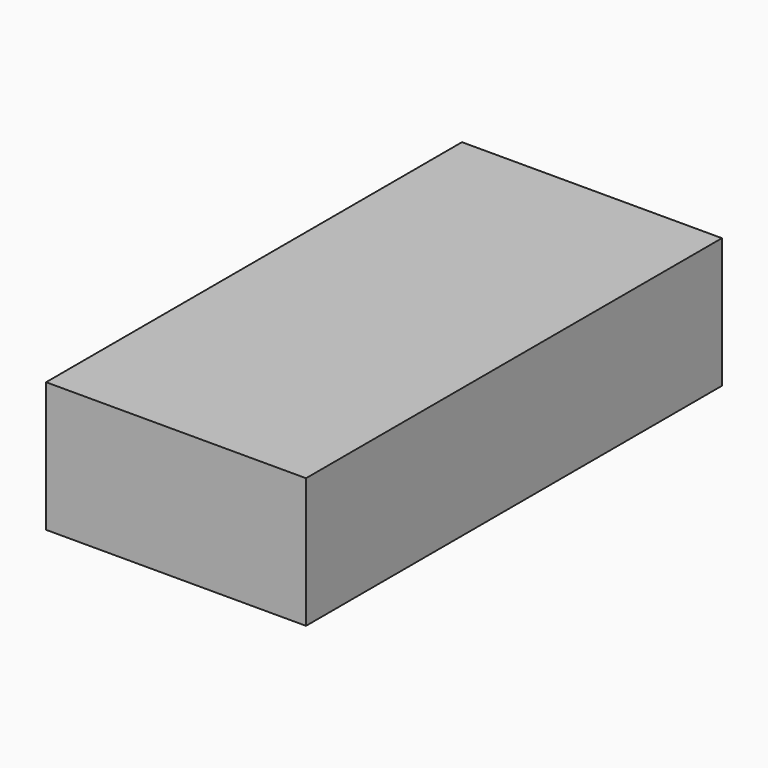
from build123d import *

# Parameters (mm, degrees)
F0_W          = 100
F0_H          = 50
F1_DEPTH      = 50
F1_DEPTH_BACK = 150


# Not quite as in the source:
# - the program builds the solid bodies; features that only make, move or delete a surface that nothing else refers to are left out


with BuildPart() as f1:
    # F0 (on Front) → F1 (new body, two sides)
    with BuildSketch(Plane.XZ) as f1_sk:
        Rectangle(F0_W, F0_H)
    extrude(amount=F1_DEPTH)
    extrude(f1_sk.sketch, amount=-F1_DEPTH_BACK)


solid = f1.part
